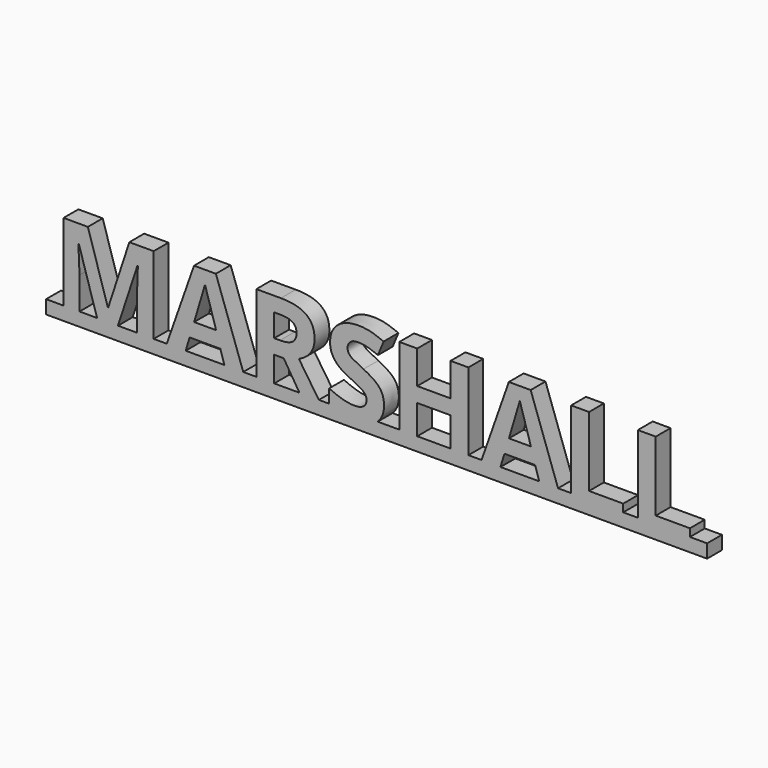
from build123d import *

# Parameters (mm, degrees)
F1_W         = 14.5061458461
F1_H         = 0.296379978
F2_DEPTH     = 0.4064
F0_TEXT_SIZE = 2.5912082896
F3_DEPTH     = 0.4064


# Not quite as in the source:
# - Text() gives the source's letters only with a copy of the font that has no kerning and outlines rounded to 1/6400 em; it was checked with that copy


with BuildPart() as f2:
    # F1 (on Front) → F2 (new body)
    with BuildSketch(Plane.XZ):
        with Locations((-2.6545238215, 0.0069378802)):
            Rectangle(F1_W, F1_H)
    extrude(amount=F2_DEPTH)

    # F0 (on Front) → F3 (join)
    with BuildSketch(Plane.XZ):
        with Locations((-9.7572168746, 0)):
            Text('MARSHALL', F0_TEXT_SIZE, font='Open Sans', font_style=FontStyle.BOLD, text_align=(TextAlign.LEFT, TextAlign.BOTTOM))
    extrude(amount=F3_DEPTH)


solid = f2.part
